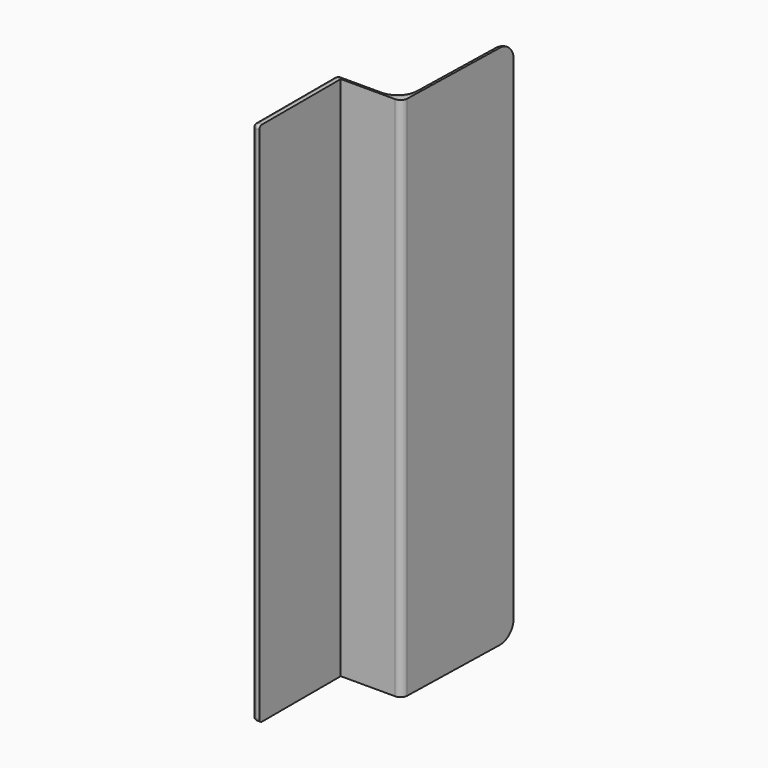
from build123d import *

# Parameters (mm, degrees)
F1_DEPTH     = 155
F2_R         = 5
F3_T1_DEPTH  = 145
F3_T3_DEPTH  = 28.172866076
F3_T5_DEPTH  = 18.1728662684
F3_T8_ANGLE  = 90
F3_T10_ANGLE = 90
F3_T12_ANGLE = 88.5674563985
F3_T14_ANGLE = 88.5674563985
F4_R         = 2
F5_R         = 1
F6_R         = 1


# Not quite as in the source:
# - a fillet or chamfer that OpenCascade refuses, or shapes differently, is made with other operations: its cross-section is extruded or revolved along the edge and cut away or added


with BuildPart() as f1:
    # F0 (on Top) → F1 (new body)
    with BuildSketch(Plane.XY):
        Polygon((-2.000000095, 0), (0, 0), (0, 30), (18, 30), (18.999999905, 69.9874980486), (17.0006250026, 70.0374980439), (16.0493903369, 32.000000095), (-2.000000095, 32.000000095), align=None)
    extrude(amount=F1_DEPTH)

    # F2
    f2_edges = [f1.edges().sort_by_distance(p)[0] for p in [
        (16.04939, 32, 77.5),
        (18.000312, 70.012498, 155),
        (18.000312, 70.012498, 0),
    ]]
    fillet(f2_edges, radius=F2_R)

    # F3: fillet of radius 2 on 6 edges, made by hand

    # F3_s2 → F3_t1 (cut)
    with BuildSketch(Plane.XY.offset(5)):
        with BuildLine():
            ThreePointArc((18.999999905, 69.9874980486), (17.5715836938, 69.4372500336), (16.9506250073, 68.0381231415))
            Line((16.9506250073, 68.0381231415), (17.0006250026, 70.0374980439))
            Line((17.0006250026, 70.0374980439), (18.999999905, 69.9874980486))
        make_face()
    extrude(amount=F3_T1_DEPTH, mode=Mode.SUBTRACT)

    # F3_s4 → F3_t3 (cut)
    with BuildSketch(Plane(origin=(1.6360154319, 65.4201701064, 0), x_dir=(0, 0, 1), z_dir=(-0.0249999976, -0.9996874512, 0))):
        with BuildLine():
            ThreePointArc((0, -17.2443741931), (0.5857864376, -15.8301606308), (2, -15.2443741931))
            Line((2, -15.2443741931), (0, -15.2443741931))
            Line((0, -15.2443741931), (0, -17.2443741931))
        make_face()
        with BuildLine():
            ThreePointArc((155, -17.2443741931), (154.4142135624, -15.8301606308), (153, -15.2443741931))
            Line((153, -15.2443741931), (155, -15.2443741931))
            Line((155, -15.2443741931), (155, -17.2443741931))
        make_face()
    extrude(amount=F3_T3_DEPTH, mode=Mode.SUBTRACT)

    # F3_s6 → F3_t5 (cut)
    with BuildSketch(Plane.YZ.offset(-7.000000095)):
        with BuildLine():
            ThreePointArc((30.000000095, 155), (31.4142136574, 154.4142135624), (32.000000095, 153))
            Line((32.000000095, 153), (32.000000095, 155))
            Line((32.000000095, 155), (30.000000095, 155))
        make_face()
        with BuildLine():
            ThreePointArc((30.000000095, 0), (31.4142136574, 0.5857864376), (32.000000095, 2))
            Line((32.000000095, 2), (32.000000095, 0))
            Line((32.000000095, 0), (30.000000095, 0))
        make_face()
    extrude(amount=F3_T5_DEPTH, mode=Mode.SUBTRACT)

    # F3_s7 → F3_t8 (revolve, cut)
    with BuildSketch(Plane.XY.offset(5)):
        with BuildLine():
            ThreePointArc((18.999999905, 69.9874980486), (17.5715836938, 69.4372500336), (16.9506250073, 68.0381231415))
            Line((16.9506250073, 68.0381231415), (17.0006250026, 70.0374980439))
            Line((17.0006250026, 70.0374980439), (18.999999905, 69.9874980486))
        make_face()
    revolve(axis=Axis((16.8756250144, 65.0390607878, 5), (-0.9996874512, 0.0249999976, 0)), revolution_arc=F3_T8_ANGLE, mode=Mode.SUBTRACT)

    # F3_s9 → F3_t10 (revolve, cut)
    with BuildSketch(Plane.XY.offset(150)):
        with BuildLine():
            ThreePointArc((18.999999905, 69.9874980486), (17.5715836938, 69.4372500336), (16.9506250073, 68.0381231415))
            Line((16.9506250073, 68.0381231415), (17.0006250026, 70.0374980439))
            Line((17.0006250026, 70.0374980439), (18.999999905, 69.9874980486))
        make_face()
    revolve(axis=Axis((16.8756250144, 65.0390607878, 150), (0.9996874512, -0.0249999976, 0)), revolution_arc=F3_T10_ANGLE, mode=Mode.SUBTRACT)

    # F3_s11 → F3_t12 (revolve, cut)
    with BuildSketch(Plane(origin=(0.9316938469, 37.2561094255, 0), x_dir=(0, 0, 1), z_dir=(0.0249999976, 0.9996874512, 0))):
        with BuildLine():
            ThreePointArc((155, 17.2443741931), (154.4142135624, 15.8301606308), (153, 15.2443741931))
            Line((153, 15.2443741931), (155, 15.2443741931))
            Line((155, 15.2443741931), (155, 17.2443741931))
        make_face()
    revolve(axis=Axis((11.1728661734, 37.000000095, 155), (0, 0, -1)), revolution_arc=F3_T12_ANGLE, mode=Mode.SUBTRACT)

    # F3_s13 → F3_t14 (revolve, cut)
    with BuildSketch(Plane(origin=(0.9316938469, 37.2561094255, 0), x_dir=(0, 0, 1), z_dir=(0.0249999976, 0.9996874512, 0))):
        with BuildLine():
            ThreePointArc((0, 17.2443741931), (0.5857864376, 15.8301606308), (2, 15.2443741931))
            Line((2, 15.2443741931), (0, 15.2443741931))
            Line((0, 15.2443741931), (0, 17.2443741931))
        make_face()
    revolve(axis=Axis((11.1728661734, 37.000000095, 0), (0, 0, -1)), revolution_arc=F3_T14_ANGLE, mode=Mode.SUBTRACT)

    # F4
    f4_edges = [f1.edges().sort_by_distance(p)[0] for p in [
        (18, 30, 77.5),
    ]]
    fillet(f4_edges, radius=F4_R)

    # F5
    f5_edges = [f1.edges().sort_by_distance(p)[0] for p in [
        (-2, 0, 77.5),
    ]]
    fillet(f5_edges, radius=F5_R)

    # F6
    f6_edges = [f1.edges().sort_by_distance(p)[0] for p in [
        (-2, 32, 77.5),
        (-0.5, 0, 0),
        (-1.707107, 0.292893, 0),
        (-2, 15.5, 0),
        (-0.5, 0, 155),
        (-1.707107, 0.292893, 155),
        (-2, 31.414214, 0.585786),
        (-2, 15.5, 155),
        (-2, 31.414214, 154.414214),
    ]]
    fillet(f6_edges, radius=F6_R)


solid = f1.part
